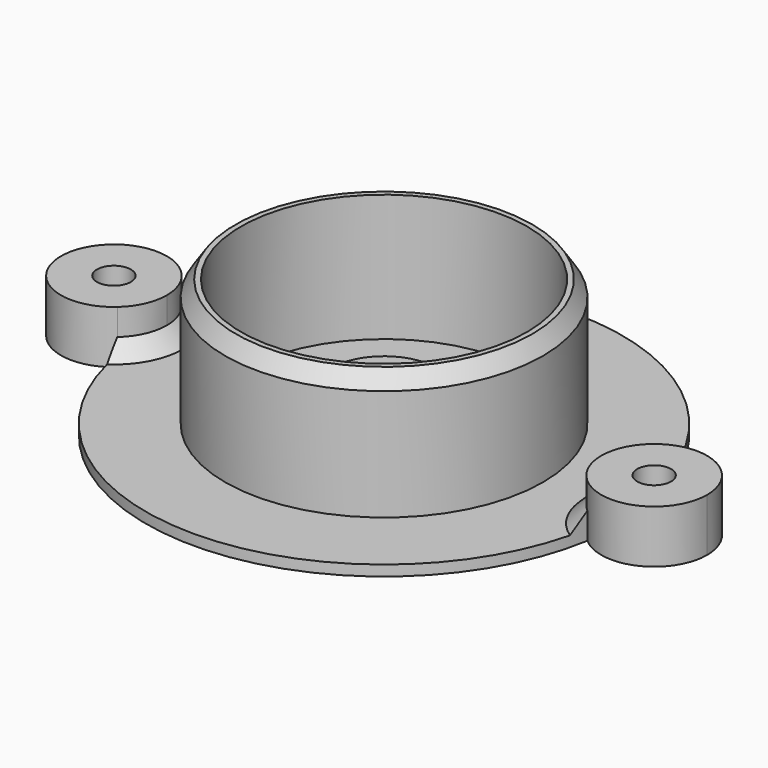
from build123d import *

# Parameters (mm, degrees)
F0_R         = 1.6
F1_DEPTH     = 5
F2_DEPTH     = 1
F3_R         = 15
F3_R_2       = 13.5
F4_DEPTH     = 12
F5_SIZE2     = 1.5
F5_SIZE      = 1
F8_T4_ANGLE  = 185.4300536725
F8_S5_R      = 22.5
F8_T6_DEPTH  = 9
F8_T10_ANGLE = 185.4300536725
F8_S11_R     = 22.5
F8_T12_DEPTH = 9
F9_R         = 5
F10_DEPTH    = 3
F11_R        = 3.25
F12_DEPTH    = 5


# Not quite as in the source:
# - a fillet or chamfer that OpenCascade refuses, or shapes differently, is made with other operations: its cross-section is extruded or revolved along the edge and cut away or added
# - a feature of the source that left no trace in its solid (it failed there, or was rolled back) is left out


with BuildPart() as f1:
    # F0 (on Top) → F1 (new body)
    with BuildSketch(Plane.XY):
        with BuildLine():
            ThreePointArc((-22.1862745098, -3.7442253372), (-22.5, 0), (-22.1862745098, 3.7442253372))
            ThreePointArc((-22.1862745098, 3.7442253372), (-30.5, 0), (-22.1862745098, -3.7442253372))
        make_face()
        with Locations((-25.5, 0)):
            Circle(F0_R, mode=Mode.SUBTRACT)
        with BuildLine():
            ThreePointArc((-20.5, 0), (-20.9410183456, 2.0532136456), (-22.1862745098, 3.7442253372))
            ThreePointArc((-22.1862745098, 3.7442253372), (-22.5, 0), (-22.1862745098, -3.7442253372))
            ThreePointArc((-22.1862745098, -3.7442253372), (-20.9410183456, -2.0532136456), (-20.5, 0))
        make_face()
    extrude(amount=F1_DEPTH)



with BuildPart() as f1b:
    # F0 (on Top) → F1, piece 2 (new body)
    with BuildSketch(Plane.XY):
        with BuildLine():
            ThreePointArc((22.1862745098, 3.7442253372), (22.4214314493, 1.8786728733), (22.5, 0))
            ThreePointArc((22.5, 0), (22.4214314493, -1.8786728733), (22.1862745098, -3.7442253372))
            ThreePointArc((22.1862745098, -3.7442253372), (27.5532136456, -4.5589816544), (30.5, 0))
            ThreePointArc((30.5, 0), (27.5532136456, 4.5589816544), (22.1862745098, 3.7442253372))
        make_face()
        with Locations((25.5, 0)):
            Circle(F0_R, mode=Mode.SUBTRACT)
        with BuildLine():
            ThreePointArc((22.1862745098, -3.7442253372), (22.4214314493, -1.8786728733), (22.5, 0))
            ThreePointArc((22.5, 0), (22.4214314493, 1.8786728733), (22.1862745098, 3.7442253372))
            ThreePointArc((22.1862745098, 3.7442253372), (20.5, 0), (22.1862745098, -3.7442253372))
        make_face()
    extrude(amount=F1_DEPTH)


with BuildPart() as f1_1:
    add(f1.part)

    add(f1b.part)  # F2 merges F1b
    # F0 (on Top) → F2 (join)
    with BuildSketch(Plane.XY):
        with BuildLine():
            ThreePointArc((22.1862745098, -3.7442253372), (20.5, 0), (22.1862745098, 3.7442253372))
            ThreePointArc((22.1862745098, 3.7442253372), (0, 22.5), (-22.1862745098, 3.7442253372))
            ThreePointArc((-22.1862745098, 3.7442253372), (-20.9410183456, 2.0532136456), (-20.5, 0))
            ThreePointArc((-20.5, 0), (-20.9410183456, -2.0532136456), (-22.1862745098, -3.7442253372))
            ThreePointArc((-22.1862745098, -3.7442253372), (0, -22.5), (22.1862745098, -3.7442253372))
        make_face()
    extrude(amount=F2_DEPTH)

    # F3 (on face) → F4 (join)
    with BuildSketch(Plane.XY.offset(1)):
        Circle(F3_R)
        Circle(F3_R_2, mode=Mode.SUBTRACT)
    extrude(amount=F4_DEPTH)

    # F5
    f5_edges = [f1_1.edges().sort_by_distance(p)[0] for p in [
        (-15, 0, 13),
    ]]
    f5_side = f1_1.faces().sort_by_distance((-14.575736, 0, 13))[0]
    chamfer(f5_edges, length=F5_SIZE, length2=F5_SIZE2, reference=f5_side)

    # F8: chamfer of 1.5 on 2 edges, made by hand


with BuildPart() as f8_tool2:
    # F8_s3 → F8_t4 (revolve)
    with BuildSketch(Plane(origin=(25.4427839223, 1.2065389767, 0), x_dir=(0, 0, 1), z_dir=(0.9988774861, 0.0473684257, 0))):
        Polygon((1, 7.7078948555), (2.5, 6.2078948555), (1, 6.2078948555), align=None)
    revolve(axis=Axis((25.5, 0, 1), (0, 0, -1)), revolution_arc=F8_T4_ANGLE)

    # F8_s5 → F8_t6 (intersect, symmetric)
    with BuildSketch(Plane.XY.offset(1.8)):
        Circle(F8_S5_R)
    extrude(amount=F8_T6_DEPTH, both=True, mode=Mode.INTERSECT)


with BuildPart() as f1_2:
    add(f1_1.part)

    # F8_t1: union F8_tool2
    add(f8_tool2.part)


with BuildPart() as f8_tool8:
    # F8_s9 → F8_t10 (revolve)
    with BuildSketch(Plane(origin=(-25.4427839223, 1.2065389767, 0), x_dir=(0, 0, 1), z_dir=(-0.9988774861, 0.0473684257, 0))):
        Polygon((1, -7.7078948555), (2.5, -6.2078948555), (1, -6.2078948555), align=None)
    revolve(axis=Axis((-25.5, 0, 1), (0, 0, 1)), revolution_arc=F8_T10_ANGLE)

    # F8_s11 → F8_t12 (intersect, symmetric)
    with BuildSketch(Plane.XY.offset(1.7)):
        Circle(F8_S11_R)
    extrude(amount=F8_T12_DEPTH, both=True, mode=Mode.INTERSECT)


with BuildPart() as f1_3:
    add(f1_2.part)

    # F8_t7: union F8_tool8
    add(f8_tool8.part)

    # F9 (on face) → F10 (join)
    with BuildSketch(Plane.XY.offset(1)):
        Circle(F9_R)
    extrude(amount=F10_DEPTH)

    # F11 (on face) → F12 (cut)
    with BuildSketch(Plane.XY.offset(4)):
        Circle(F11_R)
    extrude(amount=-F12_DEPTH, mode=Mode.SUBTRACT)


solid = f1_3.part
